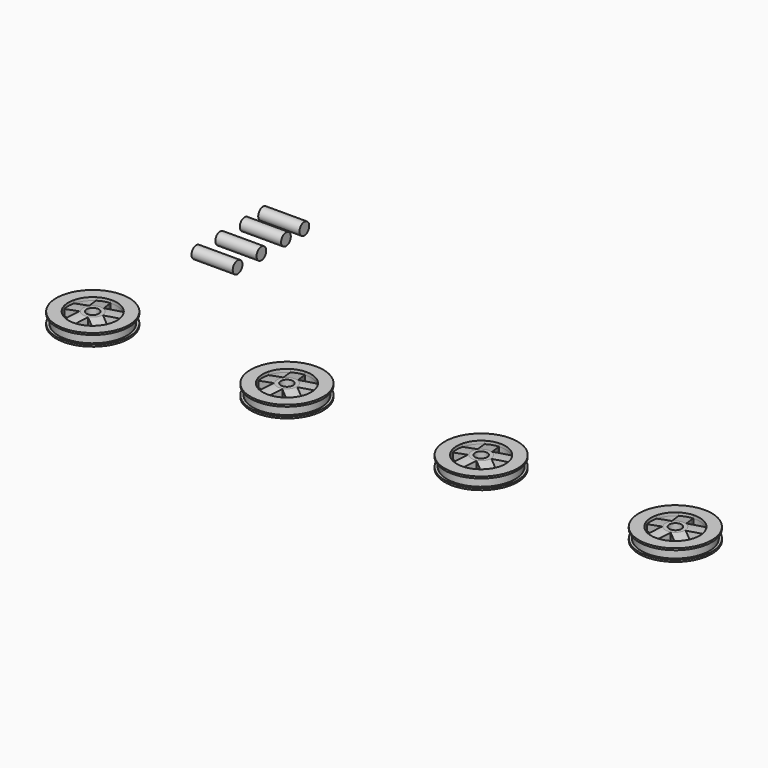
from build123d import *

# Parameters (mm, degrees)
F0_W     = 1.27
F0_H     = 2.2225
F0_W_2   = 7.62
F0_H_2   = 1.5875
F3_DEPTH = 25.4
F8_R     = 3.175
F9_DEPTH = 21.59


# Not quite as in the source:
# - after a boolean that leaves OpenCascade's solid faulty, fix() repairs it


with BuildPart() as f1:
    # F0 (on Front) → F1 (revolve)
    with BuildSketch(Plane.XZ):
        with Locations((-59.9352485356, 1.11125)):
            Rectangle(F0_W, F0_H)
        with Locations((-59.9352485356, 3.33375)):
            Rectangle(F0_W, F0_H)
        Polygon((-22.4702485356, 5.3975), (-28.8202485356, 5.3975), (-28.8202485356, 3.81), (-28.8202485356, 2.2225), (-22.4702485356, 2.2225), align=None)
        with Locations((-32.6302485356, 3.01625)):
            Rectangle(F0_W_2, F0_H_2)
        Polygon((-36.4402485356, 3.81), (-28.8202485356, 3.81), (-36.4402485356, 5.3975), align=None)
        Polygon((-22.4702485356, -0.9525), (-22.4702485356, 2.2225), (-28.8202485356, 2.2225), (-28.8202485356, 0.635), (-28.8202485356, -0.9525), align=None)
        with Locations((-32.6302485356, 1.42875)):
            Rectangle(F0_W_2, F0_H_2)
        Polygon((-36.4402485356, 2.2225), (-36.4402485356, 3.81), (-36.4402485356, 5.3975), (-38.3452485356, 5.3975), (-38.3452485356, 2.2225), align=None)
        Polygon((-36.4402485356, -0.9525), (-28.8202485356, 0.635), (-36.4402485356, 0.635), align=None)
        Polygon((-36.4402485356, 0.635), (-36.4402485356, 2.2225), (-38.3452485356, 2.2225), (-38.3452485356, -0.9525), (-36.4402485356, -0.9525), align=None)
    revolve(axis=Axis((-41.5202485356, 0, 2.0941267129), (0, 0, 1)))

    add(f1.part.fix(), mode=Mode.REPLACE)

    # F2 (on face) → F3 (cut)
    with BuildSketch(Plane.XY.offset(5.3975)):
        with BuildLine():
            Line((-41.7123280121, 10.8656756712), (-34.9781690591, 8.6776147898))
            Line((-34.9781690591, 8.6776147898), (-33.438209538, 9.7964608733))
            ThreePointArc((-33.438209538, 9.7964608733), (-37.595732707, 12.0784177569), (-42.3005402078, 12.6760066624))
            Line((-42.3005402078, 12.6760066624), (-41.7123280121, 10.8656756712))
        make_face()
        Polygon((-39.8510522546, 5.1372579143), (-34.9781690591, 8.6776147898), (-41.7123280121, 10.8656756712), align=None)
        with BuildLine():
            Line((-51.9134760092, 3.175), (-47.7515368906, 8.9034177569))
            Line((-47.7515368906, 8.9034177569), (-48.3397490863, 10.7137487482))
            ThreePointArc((-48.3397490863, 10.7137487482), (-51.7947643642, 7.4648727041), (-53.8169706598, 3.175))
            Line((-53.8169706598, 3.175), (-51.9134760092, 3.175))
        make_face()
        Polygon((-45.8902611331, 3.175), (-47.7515368906, 8.9034177569), (-51.9134760092, 3.175), align=None)
        with BuildLine():
            Line((-48.3397490863, -10.7137487482), (-47.7515368906, -8.9034177569))
            Line((-47.7515368906, -8.9034177569), (-51.9134760092, -3.175))
            Line((-51.9134760092, -3.175), (-53.8169706598, -3.175))
            ThreePointArc((-53.8169706598, -3.175), (-51.7947643642, -7.4648727041), (-48.3397490863, -10.7137487482))
        make_face()
        Polygon((-51.9134760092, -3.175), (-47.7515368906, -8.9034177569), (-45.8902611331, -3.175), align=None)
        Polygon((-41.7123280121, -10.8656756712), (-34.9781690591, -8.6776147898), (-39.8510522546, -5.1372579143), align=None)
        with BuildLine():
            Line((-33.438209538, -9.7964608733), (-34.9781690591, -8.6776147898))
            Line((-34.9781690591, -8.6776147898), (-41.7123280121, -10.8656756712))
            Line((-41.7123280121, -10.8656756712), (-42.3005402078, -12.6760066624))
            ThreePointArc((-42.3005402078, -12.6760066624), (-37.595732707, -12.0784177569), (-33.438209538, -9.7964608733))
        make_face()
        Polygon((-31.245732707, -3.5403568756), (-31.245732707, 3.5403568756), (-36.1186159026, 0), align=None)
        with BuildLine():
            Line((-29.705773186, 4.659202959), (-31.245732707, 3.5403568756))
            Line((-31.245732707, 3.5403568756), (-31.245732707, -3.5403568756))
            Line((-31.245732707, -3.5403568756), (-29.705773186, -4.659202959))
            ThreePointArc((-29.705773186, -4.659202959), (-29.0435935965, -2.3713037616), (-28.8202485356, 0))
            ThreePointArc((-28.8202485356, 0), (-29.0435935965, 2.3713037616), (-29.705773186, 4.659202959))
        make_face()
    extrude(amount=-F3_DEPTH, mode=Mode.SUBTRACT)

    # F0 (on Front) → F4 (revolve, cut)
    with BuildSketch(Plane.XZ):
        with Locations((-59.9352485356, 3.33375)):
            Rectangle(F0_W, F0_H)
        with Locations((-59.9352485356, 1.11125)):
            Rectangle(F0_W, F0_H)
    revolve(axis=Axis((-41.5202485356, 0, 2.0941267129), (0, 0, 1)), mode=Mode.SUBTRACT)

    add(f1.part.fix(), mode=Mode.REPLACE)


with BuildPart() as f5_1:
    # F5: copy of F1
    add(f1.part.moved(Location((101.6, 0, 0))))


with BuildPart() as f6_1:
    # F6: copy of F5_1
    add(f5_1.part.moved(Location((101.6, 0, 0))))


with BuildPart() as f7_1:
    # F7: copy of F6_1
    add(f6_1.part.moved(Location((101.6, 0, 0))))


with BuildPart() as f9:
    # F8 (on Right) → F9 (new body)
    with BuildSketch(Plane.YZ):
        with Locations((15.8393198696, 39.8589968681)):
            Circle(F8_R)
    extrude(amount=F9_DEPTH)


with BuildPart() as f9b:
    # F8 (on Right) → F9, piece 2 (new body)
    with BuildSketch(Plane.YZ):
        with BuildLine():
            ThreePointArc((28.2400496732, 39.8589968681), (31.4150496732, 36.6839968681), (34.5900496732, 39.8589968681))
            Line((34.5900496732, 39.8589968681), (28.2400496732, 39.8589968681))
        make_face()
        with BuildLine():
            Line((28.2400496732, 39.8589968681), (34.5900496732, 39.8589968681))
            ThreePointArc((34.5900496732, 39.8589968681), (31.4150496732, 43.0339968681), (28.2400496732, 39.8589968681))
        make_face()
    extrude(amount=F9_DEPTH)


with BuildPart() as f9c:
    # F8 (on Right) → F9, piece 3 (new body)
    with BuildSketch(Plane.YZ):
        with BuildLine():
            ThreePointArc((44.2877728855, 39.8589968681), (47.4627728855, 36.6839968681), (50.6377728855, 39.8589968681))
            Line((50.6377728855, 39.8589968681), (44.2877728855, 39.8589968681))
        make_face()
        with BuildLine():
            Line((44.2877728855, 39.8589968681), (50.6377728855, 39.8589968681))
            ThreePointArc((50.6377728855, 39.8589968681), (47.4627728855, 43.0339968681), (44.2877728855, 39.8589968681))
        make_face()
    extrude(amount=F9_DEPTH)


with BuildPart() as f9d:
    # F8 (on Right) → F9, piece 4 (new body)
    with BuildSketch(Plane.YZ):
        with BuildLine():
            ThreePointArc((62.6735622841, 39.8589968681), (59.4985622841, 43.0339968681), (56.3235622841, 39.8589968681))
            ThreePointArc((56.3235622841, 39.8589968681), (59.4985622841, 36.6839968681), (62.6735622841, 39.8589968681))
        make_face()
    extrude(amount=F9_DEPTH)


solid = Compound([f1.part, f5_1.part, f6_1.part, f7_1.part, f9.part, f9b.part, f9c.part, f9d.part])
